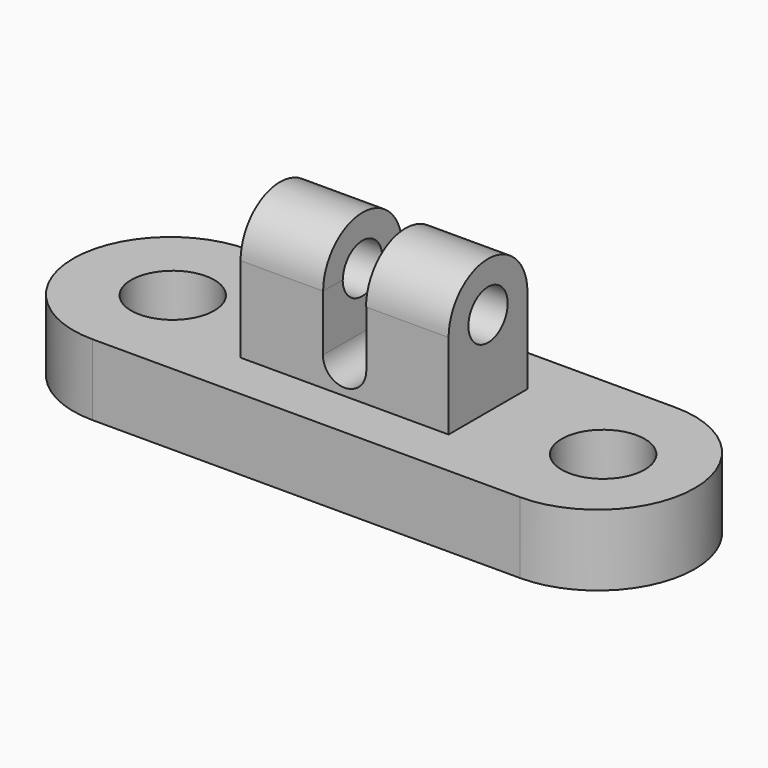
from build123d import *

# Parameters (mm, degrees)
F0_W      = 150.0394791365
F0_H      = 68.2500004768
F1_DEPTH  = 25
F2_R      = 14.6010069538
F2_R_2    = 14.601
F3_DEPTH  = 86
F4_W      = 73.0581060052
F4_H      = 34.6081331372
F5_DEPTH  = 30
F7_DEPTH  = 50
F9_DEPTH  = 29
F11_DEPTH = 29
F12_R     = 8.621691767
F13_DEPTH = 110.5


# Not quite as in the source:
# - a feature names something its author has since deleted; it is built from what else it names


with BuildPart() as f1:
    # F0 (on Top) → F1 (new body)
    with BuildSketch(Plane.XY):
        Rectangle(F0_W, F0_H)
        with BuildLine():
            Line((-75.0197395682, -34.1250002384), (-75.0197395682, 34.1250002384))
            ThreePointArc((-75.0197395682, 34.1250002384), (-109.1447398067, 0), (-75.0197395682, -34.1250002384))
        make_face()
        with BuildLine():
            ThreePointArc((75.0197395682, -34.1250002384), (109.1447398067, 0), (75.0197395682, 34.1250002384))
            Line((75.0197395682, 34.1250002384), (75.0197395682, -34.1250002384))
        make_face()
    extrude(amount=F1_DEPTH)

    # F2 (on Top) → F3 (cut)
    with BuildSketch(Plane.XY):
        with Locations((-74.1907954216, 0)):
            Circle(F2_R)
        with Locations((76.9539475441, 0)):
            Circle(F2_R_2)
    extrude(amount=F3_DEPTH, mode=Mode.SUBTRACT)

    # F4 (on face) → F5 (join)
    with BuildSketch(Plane.XY.offset(25)):
        Rectangle(F4_W, F4_H)
    extrude(amount=F5_DEPTH)

    # F6 (on face) → F7 (cut)
    with BuildSketch(Plane(origin=(0, 17.3040665686, 0), x_dir=(-1, 0, 0), z_dir=(0, 1, 0))):
        with BuildLine():
            ThreePointArc((-7.6186316787, 35.1906841607), (0, 27.572052482), (7.6186316787, 35.1906841607))
            Line((7.6186316787, 35.1906841607), (-7.6186316787, 35.1906841607))
        make_face()
        with BuildLine():
            Line((-7.6186316787, 35.1906841607), (7.6186316787, 35.1906841607))
            ThreePointArc((7.6186316787, 35.1906841607), (0, 42.8093158393), (-7.6186316787, 35.1906841607))
        make_face()
        with BuildLine():
            ThreePointArc((-7.6186316787, 35.1906841607), (0, 42.8093158393), (7.6186316787, 35.1906841607))
            Line((7.6186316787, 35.1906841607), (7.6186316787, 55))
            Line((7.6186316787, 55), (-7.6186316787, 55))
            Line((-7.6186316787, 55), (-7.6186316787, 35.1906841607))
        make_face()
    extrude(amount=-F7_DEPTH, mode=Mode.SUBTRACT)

    # F8 (on face) → F9 (join)
    with BuildSketch(Plane.YZ.offset(36.5290530026)):
        with BuildLine():
            Line((-17.3040665686, 55), (17.3040665686, 55))
            ThreePointArc((17.3040665686, 55), (0, 72.3040665686), (-17.3040665686, 55))
        make_face()
    extrude(amount=-F9_DEPTH)

    # F10 (on face) → F11 (join)
    with BuildSketch(Plane(origin=(-36.5290530026, 0, 0), x_dir=(0, -1, 0), z_dir=(-1, 0, 0))):
        with BuildLine():
            Line((-17.3040665686, 55), (17.3040665686, 55))
            ThreePointArc((17.3040665686, 55), (0, 72.3040665686), (-17.3040665686, 55))
        make_face()
    extrude(amount=-F11_DEPTH)

    # F12 (on face) → F13 (cut)
    with BuildSketch(Plane(origin=(-36.5290530026, 0, 0), x_dir=(0, -1, 0), z_dir=(-1, 0, 0))):
        with Locations((0, 55)):
            Circle(F12_R)
    extrude(amount=-F13_DEPTH, mode=Mode.SUBTRACT)


solid = f1.part
